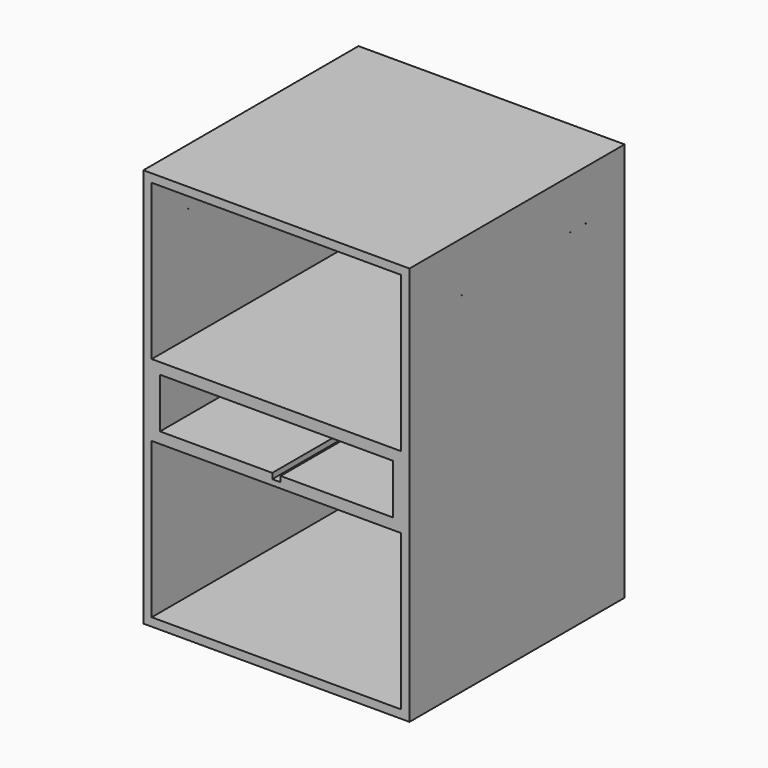
from build123d import *

# Parameters (mm, degrees)
F0_W     = 1219.2
F0_H     = 1828.8
F0_W_2   = 1143
F0_H_2   = 711.2
F0_W_3   = 1066.8
F0_H_3   = 228.6
F1_DEPTH = 609.6
F2_W     = 1219.2
F2_H     = 1828.8
F3_DEPTH = 12.7
F5_D     = 2.54
F7_D     = 2.54
F7_DEPTH = 12.7
F7_TIP   = 0.7630929862
F8_W     = 38.1
F8_H     = 1219.2
F9_DEPTH = 25.4


# Not quite as in the source:
# - a feature names something its author has since deleted; it is built from what else it names


with BuildPart() as f1:
    # F0 (on Front) → F1 (new body, symmetric)
    with BuildSketch(Plane.XZ):
        Rectangle(F0_W, F0_H)
        with Locations((0, -520.7)):
            Rectangle(F0_W_2, F0_H_2, mode=Mode.SUBTRACT)
        Rectangle(F0_W_3, F0_H_3, mode=Mode.SUBTRACT)
        with Locations((0, 520.7)):
            Rectangle(F0_W_2, F0_H_2, mode=Mode.SUBTRACT)
    extrude(amount=F1_DEPTH, both=True)

    # F2 (on face) → F3 (join)
    with BuildSketch(Plane(origin=(0, 609.6, 0), x_dir=(-1, 0, 0), z_dir=(0, 1, 0))):
        Rectangle(F2_W, F2_H)
    extrude(amount=F3_DEPTH)

    # F5 (through all)
    with Locations(Plane(origin=(-609.6, 0, 0), x_dir=(0, -1, 0), z_dir=(-1, 0, 0))):
        with Locations((-400.05, 685.8), (-311.15, 685.8), (311.15, 685.8), (400.05, 685.8)):
            Hole(F5_D / 2)

    # F7
    with Locations(Plane(origin=(0, 0, -914.4), x_dir=(1, 0, 0), z_dir=(0, 0, -1))):
        with Locations((-457.2, 457.2), (457.2, 457.2), (457.2, -457.2), (-457.2, -457.2)):
            Hole(F7_D / 2, depth=F7_DEPTH)
            with Locations((0, 0, -(F7_DEPTH + F7_TIP / 2))):  # 118° drill point
                Cone(0, F7_D / 2, F7_TIP, mode=Mode.SUBTRACT)

    # F8 (on face) → F9 (cut)
    with BuildSketch(Plane.XY.offset(-114.3)):
        Rectangle(F8_W, F8_H)
    extrude(amount=-F9_DEPTH, mode=Mode.SUBTRACT)


solid = f1.part
